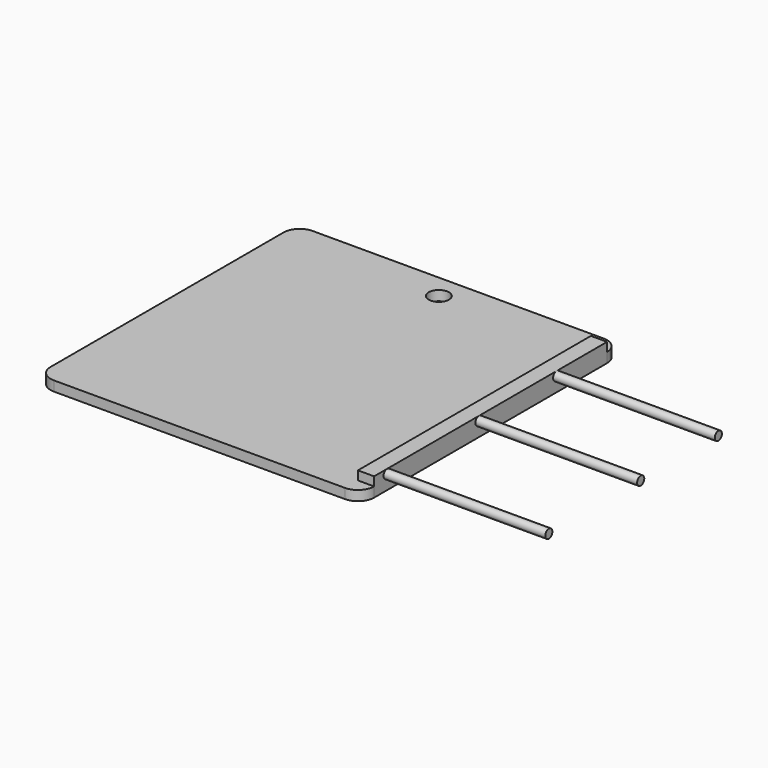
from build123d import *

# Parameters (mm, degrees)
F1_DEPTH = 1.5494
F2_R     = 1.5875
F3_DEPTH = 25.4
F5_W     = 2.54
F5_H     = 45.72
F6_DEPTH = 1.397
F7_DEPTH = 25.4


# Not quite as in the source:
# - a feature names something its author has since deleted; it is built from what else it names


with BuildPart() as f1:
    # F0 (on Top) → F1 (new body)
    with BuildSketch(Plane.XY):
        with BuildLine():
            ThreePointArc((0, 2.54), (0.7439487758, 0.7439487758), (2.54, 0))
            Line((2.54, 0), (48.26, 0))
            ThreePointArc((48.26, 0), (50.0560512242, 0.7439487758), (50.8, 2.54))
            Line((50.8, 2.54), (50.8, 48.26))
            ThreePointArc((50.8, 48.26), (50.0560512242, 50.0560512242), (48.26, 50.8))
            Line((48.26, 50.8), (2.54, 50.8))
            ThreePointArc((2.54, 50.8), (0.7439487758, 50.0560512242), (0, 48.26))
            Line((0, 48.26), (0, 2.54))
        make_face()
    extrude(amount=F1_DEPTH)

    # F2 (on face) → F3 (cut)
    with BuildSketch(Plane.XY.offset(1.5494)):
        with Locations((25.4, 46.99)):
            Circle(F2_R)
    extrude(amount=-F3_DEPTH, mode=Mode.SUBTRACT)

    # F5 (on face) → F6 (join)
    with BuildSketch(Plane.XY.offset(1.5494)):
        with Locations((49.53, 25.4)):
            Rectangle(F5_W, F5_H)
    extrude(amount=F6_DEPTH)

    # F4 (on face) → F7 (join)
    with BuildSketch(Plane.YZ.offset(50.8)):
        with BuildLine():
            ThreePointArc((5.0799999892, 1.5494), (5.5739140828, 1.7539859095), (5.7785, 2.2479))
            ThreePointArc((5.7785, 2.2479), (4.5860859172, 2.7418140905), (5.0799999892, 1.5494))
        make_face()
        with BuildLine():
            ThreePointArc((23.8125, 2.2479), (22.6200859133, 2.7418140867), (23.114, 1.5494))
            ThreePointArc((23.114, 1.5494), (23.6079140867, 1.7539859133), (23.8125, 2.2479))
        make_face()
        with BuildLine():
            ThreePointArc((39.0525, 2.2479), (37.8600859133, 2.7418140867), (38.354, 1.5494))
            ThreePointArc((38.354, 1.5494), (38.8479140867, 1.7539859133), (39.0525, 2.2479))
        make_face()
    extrude(amount=F7_DEPTH)


solid = f1.part
